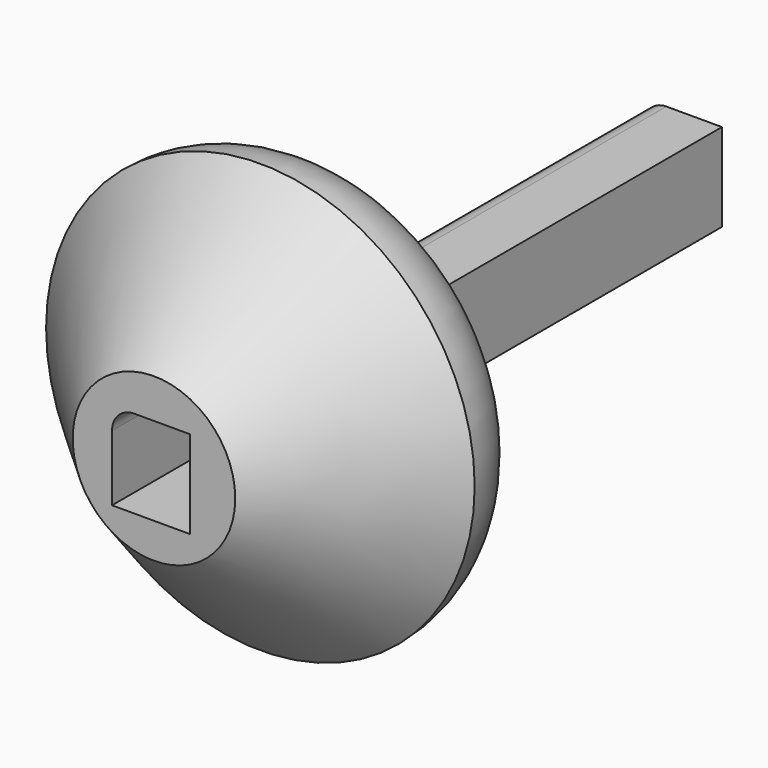
from build123d import *

# Parameters (mm, degrees)
F0_R     = 122.7600062275
F0_W     = 44.5440113544
F0_H     = 50.3597706556
F1_DEPTH = 127
F2_R     = 50.8
F3_SIZE  = 76.19999
F4_R     = 12.7
F6_DEPTH = 254


# Not quite as in the source:
# - a fillet or chamfer is up to 0.001 mm smaller than in the source, because OpenCascade refuses the exact size


with BuildPart() as f1:
    # F0 (on Front) → F1 (new body)
    with BuildSketch(Plane.XZ):
        Circle(F0_R)
        with Locations((-1.7414242029, -1.2165829539)):
            Rectangle(F0_W, F0_H, mode=Mode.SUBTRACT)
    extrude(amount=F1_DEPTH)

    # F2
    f2_edges = [f1.edges().sort_by_distance(p)[0] for p in [
        (-122.760006, 0, 0),
    ]]
    fillet(f2_edges, radius=F2_R)

    # F3 (size 76.2 in the source; OpenCascade refuses exactly that, so slightly less here)
    f3_edges = [f1.edges().sort_by_distance(p)[0] for p in [
        (-122.760006, -127, 0),
    ]]
    chamfer(f3_edges, length=F3_SIZE)

    # F4
    f4_edges = [f1.edges().sort_by_distance(p)[0] for p in [
        (-24.01343, -63.5, 23.963302),
    ]]
    fillet(f4_edges, radius=F4_R)


with BuildPart() as f6:
    # F5 (on face) → F6 (new body)
    with BuildSketch(Plane(origin=(0, 0, 0), x_dir=(-1, 0, 0), z_dir=(0, 1, 0))):
        with BuildLine():
            Line((24.0134298801, -26.3964682817), (24.0134298801, 11.2633023739))
            ThreePointArc((24.0134298801, 11.2633023739), (20.2936860012, 20.243558495), (11.3134298801, 23.9633023739))
            Line((11.3134298801, 23.9633023739), (-20.5305814743, 23.9633023739))
            Line((-20.5305814743, 23.9633023739), (-20.5305814743, -26.3964682817))
            Line((-20.5305814743, -26.3964682817), (24.0134298801, -26.3964682817))
        make_face()
    extrude(amount=F6_DEPTH)


solid = Compound([f1.part, f6.part])
